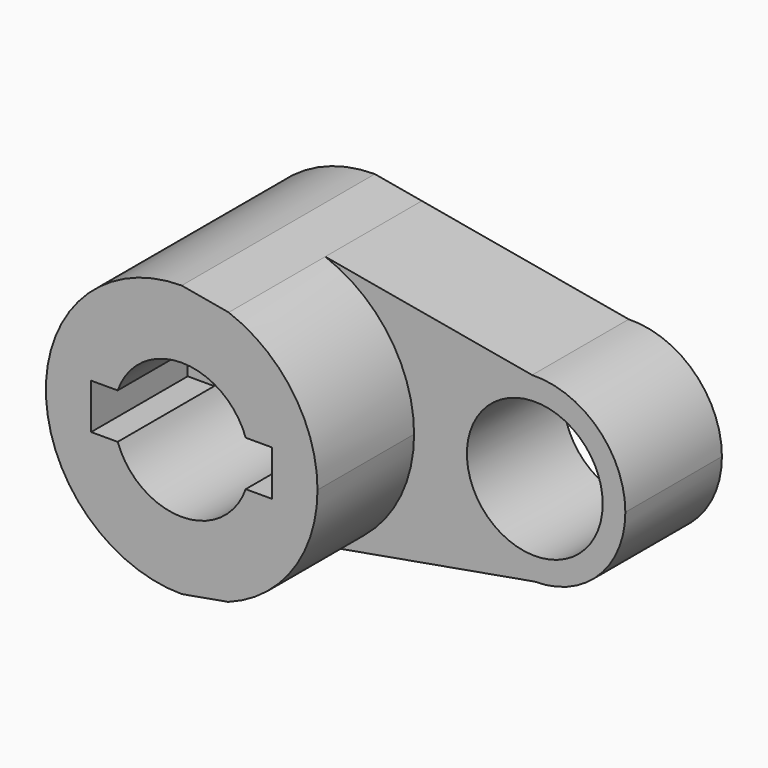
from build123d import *

# Parameters (mm, degrees)
F0_R     = 14.2875
F1_DEPTH = 25.4
F2_DEPTH = 50.8


with BuildPart() as f1:
    # F0 (on Front) → F1 (new body)
    with BuildSketch(Plane.XZ):
        with BuildLine():
            Line((9.8852824268, 26.8106660929), (0, 28.575))
            ThreePointArc((0, 28.575), (-28.575, 0), (0, -28.575))
            Line((0, -28.575), (9.7880218685, -26.8463266184))
            ThreePointArc((9.7880218685, -26.8463266184), (23.4117849586, -16.3834962707), (28.575, 0))
            ThreePointArc((28.575, 0), (23.4414437519, 16.3410323978), (9.8852824268, 26.8106660929))
        make_face()
        with BuildLine():
            ThreePointArc((-13.4703841816, 4.7625), (0, 14.2875), (13.4703841816, 4.7625))
            Line((13.4703841816, 4.7625), (19.05, 4.7625))
            Line((19.05, 4.7625), (19.05, -4.7625))
            Line((19.05, -4.7625), (13.4703841816, -4.7625))
            ThreePointArc((13.4703841816, -4.7625), (0, -14.2875), (-13.4703841816, -4.7625))
            Line((-13.4703841816, -4.7625), (-19.05, -4.7625))
            Line((-19.05, -4.7625), (-19.05, 4.7625))
            Line((-19.05, 4.7625), (-13.4703841816, 4.7625))
        make_face(mode=Mode.SUBTRACT)
        with BuildLine():
            Line((53.4134443953, 19.0417214375), (9.8852824268, 26.8106660929))
            ThreePointArc((9.8852824268, 26.8106660929), (23.4414437519, 16.3410323978), (28.575, 0))
            ThreePointArc((28.575, 0), (23.4117849586, -16.3834962707), (9.7880218685, -26.8463266184))
            Line((9.7880218685, -26.8463266184), (53.9323258703, -19.0499522025))
            ThreePointArc((53.9323258703, -19.0499522025), (34.9267671799, -0.2594733756), (53.4134443953, 19.0417214375))
        make_face()
        with BuildLine():
            ThreePointArc((73.025, 0), (67.2453591837, 13.6674821066), (53.4134443953, 19.0417214375))
            ThreePointArc((53.4134443953, 19.0417214375), (34.9267671799, -0.2594733756), (53.9323258703, -19.0499522025))
            ThreePointArc((53.9323258703, -19.0499522025), (67.4302881394, -13.4854633248), (73.025, 0))
        make_face()
        with Locations((53.975, 0)):
            Circle(F0_R, mode=Mode.SUBTRACT)
        with BuildLine():
            ThreePointArc((-13.4703841816, -4.7625), (-14.2875, 0), (-13.4703841816, 4.7625))
            Line((-13.4703841816, 4.7625), (-19.05, 4.7625))
            Line((-19.05, 4.7625), (-19.05, -4.7625))
            Line((-19.05, -4.7625), (-13.4703841816, -4.7625))
        make_face()
    extrude(amount=F1_DEPTH)

    # F0 (on Front) → F2 (join)
    with BuildSketch(Plane.XZ):
        with BuildLine():
            Line((9.8852824268, 26.8106660929), (0, 28.575))
            ThreePointArc((0, 28.575), (-28.575, 0), (0, -28.575))
            Line((0, -28.575), (9.7880218685, -26.8463266184))
            ThreePointArc((9.7880218685, -26.8463266184), (23.4117849586, -16.3834962707), (28.575, 0))
            ThreePointArc((28.575, 0), (23.4414437519, 16.3410323978), (9.8852824268, 26.8106660929))
        make_face()
        with BuildLine():
            ThreePointArc((-13.4703841816, 4.7625), (0, 14.2875), (13.4703841816, 4.7625))
            Line((13.4703841816, 4.7625), (19.05, 4.7625))
            Line((19.05, 4.7625), (19.05, -4.7625))
            Line((19.05, -4.7625), (13.4703841816, -4.7625))
            ThreePointArc((13.4703841816, -4.7625), (0, -14.2875), (-13.4703841816, -4.7625))
            Line((-13.4703841816, -4.7625), (-19.05, -4.7625))
            Line((-19.05, -4.7625), (-19.05, 4.7625))
            Line((-19.05, 4.7625), (-13.4703841816, 4.7625))
        make_face(mode=Mode.SUBTRACT)
    extrude(amount=F2_DEPTH)


solid = f1.part
